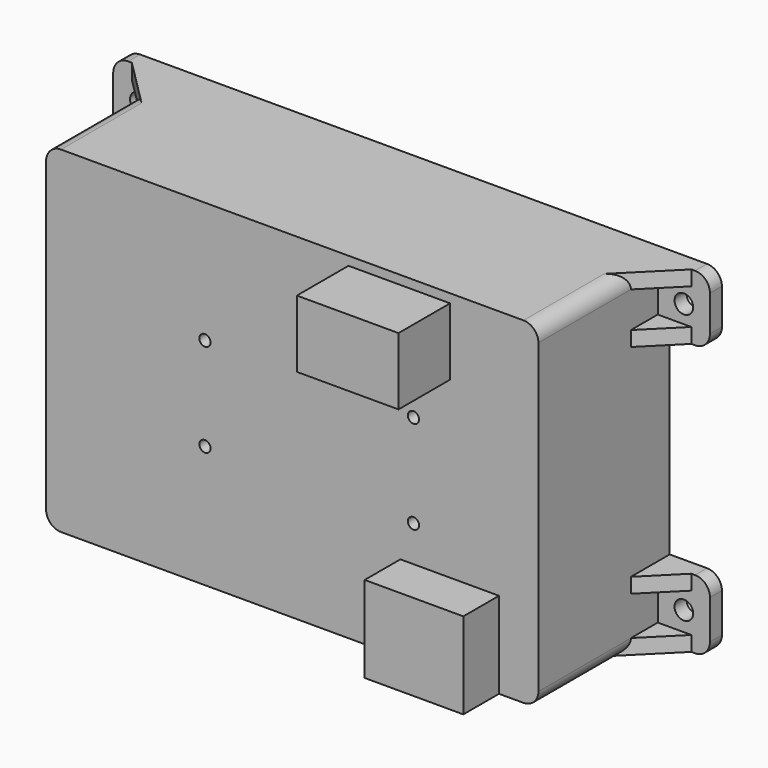
from build123d import *

# Parameters (mm, degrees)
F0_R      = 2.25
F1_DEPTH  = 66
F0_R_2    = 3.75
F2_DEPTH  = 6
F5_W      = 40.8705817536
F5_H      = 27.0229801536
F6_DEPTH  = 25.93
F5_W_2    = 39.6605432034
F5_H_2    = 34.7132187133
F7_DEPTH  = 17.926812
F8_REACH  = 45.9022057631
F9_REACH  = 45.9022057631
F10_START = 2.5
F0_R_3    = 3.5
F10_DEPTH = 8


with BuildPart() as f1:
    # F0 (on Front) → F1 (new body)
    with BuildSketch(Plane.XZ):
        with BuildLine():
            Line((85.8146208827, 61.2765278835), (-100.1853791173, 61.2765278835))
            ThreePointArc((-100.1853791173, 61.2765278835), (-104.4280198044, 59.5191685706), (-106.1853791173, 55.2765278835))
            Line((-106.1853791173, 55.2765278835), (-106.1853791173, 40.8978178835))
            Line((-106.1853791173, 40.8978178835), (-106.1853791173, 34.8978178835))
            Line((-106.1853791173, 34.8978178835), (-106.1853791173, -46.4609452256))
            Line((-106.1853791173, -46.4609452256), (-106.1853791173, -52.4609452256))
            Line((-106.1853791173, -52.4609452256), (-106.1853791173, -68.1434721165))
            ThreePointArc((-106.1853791173, -68.1434721165), (-104.4280198044, -72.3861128036), (-100.1853791173, -74.1434721165))
            Line((-100.1853791173, -74.1434721165), (-45.1853791173, -74.1434721165))
            Line((-45.1853791173, -74.1434721165), (-30.1853791173, -74.1434721165))
            Line((-30.1853791173, -74.1434721165), (85.8146208827, -74.1434721165))
            ThreePointArc((85.8146208827, -74.1434721165), (90.0572615698, -72.3861128036), (91.8146208827, -68.1434721165))
            Line((91.8146208827, -68.1434721165), (91.8146208827, -52.4609452256))
            Line((91.8146208827, -52.4609452256), (91.8146208827, -46.4609452256))
            Line((91.8146208827, -46.4609452256), (91.8146208827, 34.8978178835))
            Line((91.8146208827, 34.8978178835), (91.8146208827, 40.8978178835))
            Line((91.8146208827, 40.8978178835), (91.8146208827, 55.2765278835))
            ThreePointArc((91.8146208827, 55.2765278835), (90.0572615698, 59.5191685706), (85.8146208827, 61.2765278835))
        make_face()
        with Locations((-42.2896091173, -24.9734721165)):
            Circle(F0_R, mode=Mode.SUBTRACT)
        with Locations((41.5646208827, -24.9734721165)):
            Circle(F0_R, mode=Mode.SUBTRACT)
        with Locations((-42.2896091173, 12.5265278835)):
            Circle(F0_R, mode=Mode.SUBTRACT)
        with Locations((41.5646208827, 12.5265278835)):
            Circle(F0_R, mode=Mode.SUBTRACT)
    extrude(amount=F1_DEPTH)

    # F0 (on Front) → F2 (join)
    with BuildSketch(Plane.XZ):
        with BuildLine():
            Line((-106.1853791173, 40.8978178835), (-106.1853791173, 55.2765278835))
            Line((-106.1853791173, 55.2765278835), (-119.6853791173, 55.2765278835))
            Line((-119.6853791173, 55.2765278835), (-119.6853791173, 61.2765278835))
            Line((-119.6853791173, 61.2765278835), (-121.1853791173, 61.2765278835))
            ThreePointArc((-121.1853791173, 61.2765278835), (-125.4280198044, 59.5191685706), (-127.1853791173, 55.2765278835))
            Line((-127.1853791173, 55.2765278835), (-127.1853791173, 40.8978178835))
            ThreePointArc((-127.1853791173, 40.8978178835), (-125.4280198044, 36.6551771964), (-121.1853791173, 34.8978178835))
            Line((-121.1853791173, 34.8978178835), (-119.6853791173, 34.8978178835))
            Line((-119.6853791173, 34.8978178835), (-119.6853791173, 40.8978178835))
            Line((-119.6853791173, 40.8978178835), (-106.1853791173, 40.8978178835))
        make_face()
        with Locations((-116.6853791173, 48.0871728835)):
            Circle(F0_R_2, mode=Mode.SUBTRACT)
        with BuildLine():
            Line((106.8146208827, 61.2765278835), (105.3146208827, 61.2765278835))
            Line((105.3146208827, 61.2765278835), (105.3146208827, 55.2765278835))
            Line((105.3146208827, 55.2765278835), (91.8146208827, 55.2765278835))
            Line((91.8146208827, 55.2765278835), (91.8146208827, 40.8978178835))
            Line((91.8146208827, 40.8978178835), (105.3146208827, 40.8978178835))
            Line((105.3146208827, 40.8978178835), (105.3146208827, 34.8978178835))
            Line((105.3146208827, 34.8978178835), (106.8146208827, 34.8978178835))
            ThreePointArc((106.8146208827, 34.8978178835), (111.0572615698, 36.6551771964), (112.8146208827, 40.8978178835))
            Line((112.8146208827, 40.8978178835), (112.8146208827, 55.2765278835))
            ThreePointArc((112.8146208827, 55.2765278835), (111.0572615698, 59.5191685706), (106.8146208827, 61.2765278835))
        make_face()
        with Locations((102.3146208827, 48.0871728835)):
            Circle(F0_R_2, mode=Mode.SUBTRACT)
        with BuildLine():
            Line((105.3146208827, -52.4609452256), (91.8146208827, -52.4609452256))
            Line((91.8146208827, -52.4609452256), (91.8146208827, -68.1434721165))
            Line((91.8146208827, -68.1434721165), (105.3146208827, -68.1434721165))
            Line((105.3146208827, -68.1434721165), (105.3146208827, -74.1434721165))
            Line((105.3146208827, -74.1434721165), (106.8146208827, -74.1434721165))
            ThreePointArc((106.8146208827, -74.1434721165), (111.0572615698, -72.3861128036), (112.8146208827, -68.1434721165))
            Line((112.8146208827, -68.1434721165), (112.8146208827, -52.4609452256))
            ThreePointArc((112.8146208827, -52.4609452256), (111.0572615698, -48.2183045385), (106.8146208827, -46.4609452256))
            Line((106.8146208827, -46.4609452256), (105.3146208827, -46.4609452256))
            Line((105.3146208827, -46.4609452256), (105.3146208827, -52.4609452256))
        make_face()
        with Locations((102.3146208827, -60.302208671)):
            Circle(F0_R_2, mode=Mode.SUBTRACT)
        with BuildLine():
            Line((-106.1853791173, -68.1434721165), (-106.1853791173, -52.4609452256))
            Line((-106.1853791173, -52.4609452256), (-119.6853791173, -52.4609452256))
            Line((-119.6853791173, -52.4609452256), (-119.6853791173, -46.4609452256))
            Line((-119.6853791173, -46.4609452256), (-121.1853791173, -46.4609452256))
            ThreePointArc((-121.1853791173, -46.4609452256), (-125.4280198044, -48.2183045385), (-127.1853791173, -52.4609452256))
            Line((-127.1853791173, -52.4609452256), (-127.1853791173, -68.1434721165))
            ThreePointArc((-127.1853791173, -68.1434721165), (-125.4280198044, -72.3861128036), (-121.1853791173, -74.1434721165))
            Line((-121.1853791173, -74.1434721165), (-119.6853791173, -74.1434721165))
            Line((-119.6853791173, -74.1434721165), (-119.6853791173, -68.1434721165))
            Line((-119.6853791173, -68.1434721165), (-106.1853791173, -68.1434721165))
        make_face()
        with Locations((-116.6853791173, -60.302208671)):
            Circle(F0_R_2, mode=Mode.SUBTRACT)
        with BuildLine():
            ThreePointArc((-106.1853791173, 55.2765278835), (-104.4280198044, 59.5191685706), (-100.1853791173, 61.2765278835))
            Line((-100.1853791173, 61.2765278835), (-106.1853791173, 61.2765278835))
            Line((-106.1853791173, 61.2765278835), (-119.6853791173, 61.2765278835))
            Line((-119.6853791173, 61.2765278835), (-119.6853791173, 55.2765278835))
            Line((-119.6853791173, 55.2765278835), (-106.1853791173, 55.2765278835))
        make_face()
        Polygon((-106.1853791173, 34.8978178835), (-106.1853791173, 40.8978178835), (-119.6853791173, 40.8978178835), (-119.6853791173, 34.8978178835), (-112.1853791173, 34.8978178835), align=None)
        Polygon((-106.1853791173, -52.4609452256), (-106.1853791173, -46.4609452256), (-112.1853791173, -46.4609452256), (-119.6853791173, -46.4609452256), (-119.6853791173, -52.4609452256), align=None)
        with BuildLine():
            ThreePointArc((-100.1853791173, -74.1434721165), (-104.4280198044, -72.3861128036), (-106.1853791173, -68.1434721165))
            Line((-106.1853791173, -68.1434721165), (-119.6853791173, -68.1434721165))
            Line((-119.6853791173, -68.1434721165), (-119.6853791173, -74.1434721165))
            Line((-119.6853791173, -74.1434721165), (-100.1853791173, -74.1434721165))
        make_face()
        with BuildLine():
            Line((105.3146208827, -68.1434721165), (91.8146208827, -68.1434721165))
            ThreePointArc((91.8146208827, -68.1434721165), (90.0572615698, -72.3861128036), (85.8146208827, -74.1434721165))
            Line((85.8146208827, -74.1434721165), (105.3146208827, -74.1434721165))
            Line((105.3146208827, -74.1434721165), (105.3146208827, -68.1434721165))
        make_face()
        Polygon((97.8146208827, -46.4609452256), (91.8146208827, -46.4609452256), (91.8146208827, -52.4609452256), (105.3146208827, -52.4609452256), (105.3146208827, -46.4609452256), align=None)
        Polygon((105.3146208827, 40.8978178835), (91.8146208827, 40.8978178835), (91.8146208827, 34.8978178835), (97.8146208827, 34.8978178835), (105.3146208827, 34.8978178835), align=None)
        with BuildLine():
            Line((105.3146208827, 61.2765278835), (85.8146208827, 61.2765278835))
            ThreePointArc((85.8146208827, 61.2765278835), (90.0572615698, 59.5191685706), (91.8146208827, 55.2765278835))
            Line((91.8146208827, 55.2765278835), (105.3146208827, 55.2765278835))
            Line((105.3146208827, 55.2765278835), (105.3146208827, 61.2765278835))
        make_face()
    extrude(amount=F2_DEPTH)

    # F5 (on face) → F6 (join)
    with BuildSketch(Plane.XZ.offset(66)):
        with Locations((35.8588262461, 44.2000478506)):
            Rectangle(F5_W, F5_H)
    extrude(amount=F6_DEPTH)

    # F5 (on face) → F7 (join)
    with BuildSketch(Plane.XZ.offset(66)):
        with Locations((56.1274141073, -56.7868627598)):
            Rectangle(F5_W_2, F5_H_2)
    extrude(amount=F7_DEPTH)

    f8_end = Plane(origin=(-109.9353791173, -15.75, -4.1434721165), x_dir=(-0.7071067812, 0.7071067812, 0), z_dir=(-0.7071067812, -0.7071067812, 0))
    # F0 (on Front) → F8 (join, up to a plane its end follows)
    with BuildSketch(Plane.XZ):
        with BuildLine():
            ThreePointArc((-106.1853791173, 55.2765278835), (-104.4280198044, 59.5191685706), (-100.1853791173, 61.2765278835))
            Line((-100.1853791173, 61.2765278835), (-106.1853791173, 61.2765278835))
            Line((-106.1853791173, 61.2765278835), (-119.6853791173, 61.2765278835))
            Line((-119.6853791173, 61.2765278835), (-119.6853791173, 55.2765278835))
            Line((-119.6853791173, 55.2765278835), (-106.1853791173, 55.2765278835))
        make_face()
        Polygon((-106.1853791173, 34.8978178835), (-106.1853791173, 40.8978178835), (-119.6853791173, 40.8978178835), (-119.6853791173, 34.8978178835), (-112.1853791173, 34.8978178835), align=None)
        Polygon((-106.1853791173, -52.4609452256), (-106.1853791173, -46.4609452256), (-112.1853791173, -46.4609452256), (-119.6853791173, -46.4609452256), (-119.6853791173, -52.4609452256), align=None)
        with BuildLine():
            ThreePointArc((-100.1853791173, -74.1434721165), (-104.4280198044, -72.3861128036), (-106.1853791173, -68.1434721165))
            Line((-106.1853791173, -68.1434721165), (-119.6853791173, -68.1434721165))
            Line((-119.6853791173, -68.1434721165), (-119.6853791173, -74.1434721165))
            Line((-119.6853791173, -74.1434721165), (-100.1853791173, -74.1434721165))
        make_face()
    f8_long = extrude(amount=F8_REACH, mode=Mode.PRIVATE)
    add(split(f8_long, bisect_by=f8_end, keep=Keep.BOTTOM, mode=Mode.PRIVATE))

    f9_end = Plane(origin=(95.5646208827, -15.75, -4.1434721165), x_dir=(0.7071067812, 0.7071067812, 0), z_dir=(-0.7071067812, 0.7071067812, 0))
    # F0 (on Front) → F9 (join, up to a plane its end follows)
    with BuildSketch(Plane.XZ):
        with BuildLine():
            Line((105.3146208827, 61.2765278835), (85.8146208827, 61.2765278835))
            ThreePointArc((85.8146208827, 61.2765278835), (90.0572615698, 59.5191685706), (91.8146208827, 55.2765278835))
            Line((91.8146208827, 55.2765278835), (105.3146208827, 55.2765278835))
            Line((105.3146208827, 55.2765278835), (105.3146208827, 61.2765278835))
        make_face()
        Polygon((105.3146208827, 40.8978178835), (91.8146208827, 40.8978178835), (91.8146208827, 34.8978178835), (97.8146208827, 34.8978178835), (105.3146208827, 34.8978178835), align=None)
        Polygon((97.8146208827, -46.4609452256), (91.8146208827, -46.4609452256), (91.8146208827, -52.4609452256), (105.3146208827, -52.4609452256), (105.3146208827, -46.4609452256), align=None)
        with BuildLine():
            Line((105.3146208827, -68.1434721165), (91.8146208827, -68.1434721165))
            ThreePointArc((91.8146208827, -68.1434721165), (90.0572615698, -72.3861128036), (85.8146208827, -74.1434721165))
            Line((85.8146208827, -74.1434721165), (105.3146208827, -74.1434721165))
            Line((105.3146208827, -74.1434721165), (105.3146208827, -68.1434721165))
        make_face()
    f9_long = extrude(amount=F9_REACH, mode=Mode.PRIVATE)
    add(split(f9_long, bisect_by=f9_end, keep=Keep.TOP, mode=Mode.PRIVATE))

    # F0 (on Front) → F10 (join)
    with BuildSketch(Plane.XZ.offset(F10_START)):
        with BuildLine():
            Line((-30.1853791173, -74.1434721165), (-45.1853791173, -74.1434721165))
            Line((-45.1853791173, -74.1434721165), (-45.1853791173, -83.1434721165))
            ThreePointArc((-45.1853791173, -83.1434721165), (-43.7209130232, -86.6790060224), (-40.1853791173, -88.1434721165))
            Line((-40.1853791173, -88.1434721165), (-35.1853791173, -88.1434721165))
            ThreePointArc((-35.1853791173, -88.1434721165), (-31.6498452114, -86.6790060224), (-30.1853791173, -83.1434721165))
            Line((-30.1853791173, -83.1434721165), (-30.1853791173, -74.1434721165))
        make_face()
        with Locations((-37.6853791173, -80.6434721165)):
            Circle(F0_R_3, mode=Mode.SUBTRACT)
    extrude(amount=F10_DEPTH)


solid = f1.part
